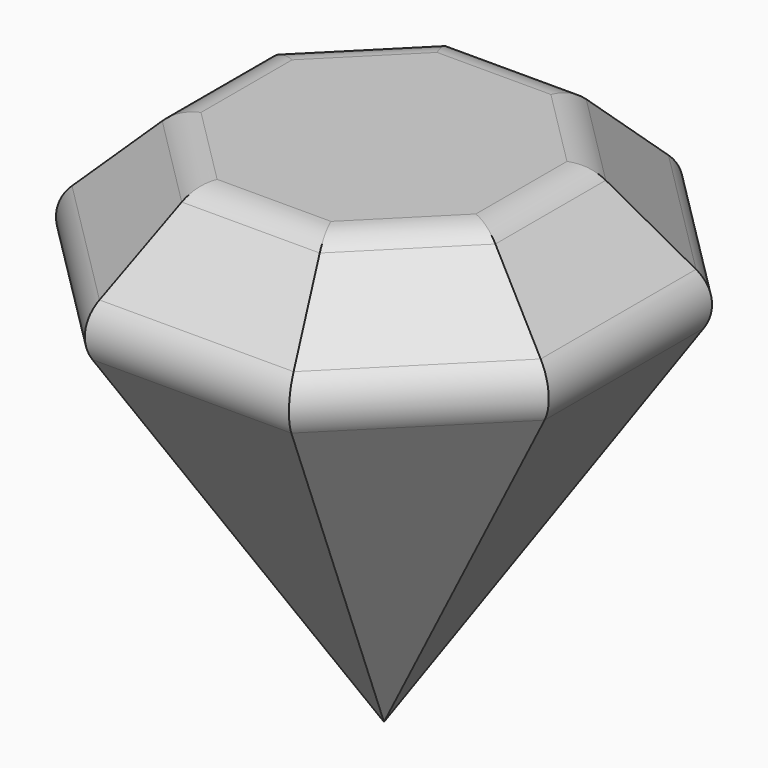
from build123d import *

# Parameters (mm, degrees)
F1_DEPTH = 12.7
F2_SIZE2 = 12.69999
F2_SIZE  = 12.69999
F6_R     = 5.08


# Not quite as in the source:
# - a fillet or chamfer is up to 0.001 mm smaller than in the source, because OpenCascade refuses the exact size


with BuildPart() as f1:
    # F0 (on Top) → F1 (new body)
    with BuildSketch(Plane.XY):
        Polygon((-31.75, 13.1512806053), (-31.75, -13.1512806053), (-13.1512806053, -31.75), (13.1512806053, -31.75), (31.75, -13.1512806053), (31.75, 13.1512806053), (13.1512806053, 31.75), (-13.1512806053, 31.75), align=None)
    extrude(amount=F1_DEPTH)

    # F2 (size 12.7 and 12.7 in the source; OpenCascade refuses exactly that, so slightly less here)
    f2_edges = [f1.edges().sort_by_distance(p)[0] for p in [
        (-22.45064, 22.45064, 12.7),
        (-31.75, 0, 12.7),
        (-22.45064, -22.45064, 12.7),
        (0, -31.75, 12.7),
        (22.45064, -22.45064, 12.7),
        (31.75, 0, 12.7),
        (22.45064, 22.45064, 12.7),
        (0, 31.75, 12.7),
    ]]
    chamfer(f2_edges, length=F2_SIZE, length2=F2_SIZE2)

    # F1_face (on face) → F5 section 0
    with BuildSketch(Plane(origin=(0, 0, 0), x_dir=(1, 0, 0), z_dir=(0, 0, -1)), mode=Mode.PRIVATE) as f5_s0:
        Polygon((-31.75, -13.1512806053), (-13.1512806053, -31.75), (13.1512806053, -31.75), (31.75, -13.1512806053), (31.75, 13.1512806053), (13.1512806053, 31.75), (-13.1512806053, 31.75), (-31.75, 13.1512806053), align=None)
    loft([f5_s0.sketch, Vertex(0, 0, -50.8)])

    # F6
    f6_edges = [f1.edges().sort_by_distance(p)[0] for p in [
        (-13.470391, 13.470391, 12.7),
        (0, 19.05001, 12.7),
        (-19.05001, 0, 12.7),
        (13.470391, 13.470391, 12.7),
        (-13.470391, -13.470391, 12.7),
        (19.05001, 0, 12.7),
        (0, -19.05001, 12.7),
        (13.470391, -13.470391, 12.7),
        (-22.45064, 22.45064, 1e-05),
        (0, 31.75, 1e-05),
        (-31.75, 0, 0),
        (22.45064, 22.45064, 0),
        (-22.45064, -22.45064, 0),
        (31.75, 0, 0),
        (0, -31.75, 0),
        (22.45064, -22.45064, 0),
    ]]
    fillet(f6_edges, radius=F6_R)


solid = f1.part
